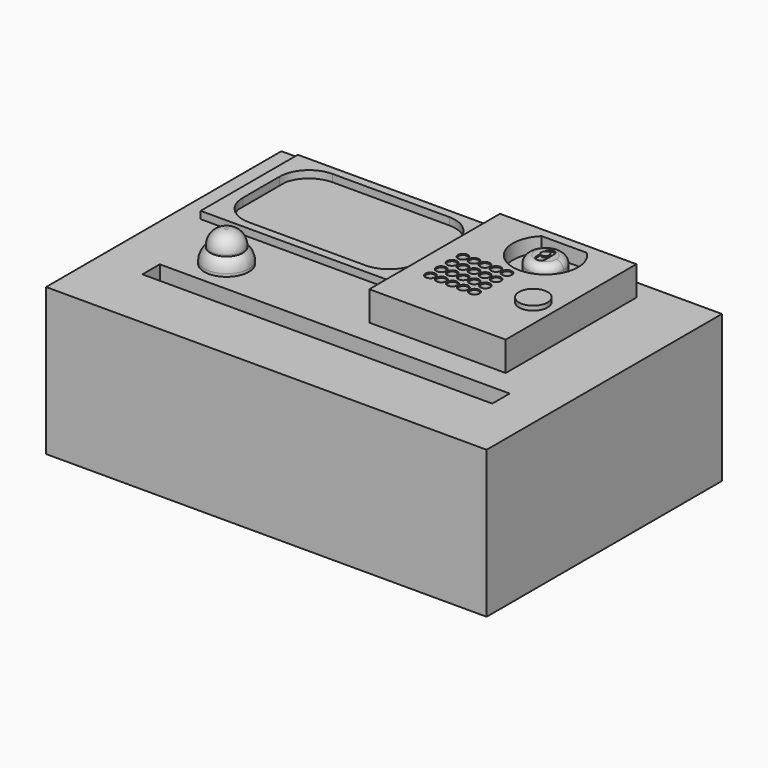
from build123d import *

# Parameters (mm, degrees)
F0_W      = 76.095610857
F0_H      = 25.4
F1_DEPTH  = 50.8
F2_W      = 60.4380872101
F2_H      = 3.7578083575
F3_DEPTH  = 63.5
F2_R      = 3.8481
F2_R_2    = 2.8067
F4_DEPTH  = 2.54
F5_DEPTH  = 5.334
F2_W_2    = 23.5645882785
F2_H_2    = 28.2227061689
F7_DEPTH  = 5.08
F8_R      = 0.7366
F8_R_2    = 0.7422011714
F8_R_3    = 0.7366978513
F9_DEPTH  = 1.1684
F10_SIZE  = 0.127
F8_R_4    = 2.4687366623
F11_DEPTH = 0.762
F12_DEPTH = 2.54
F13_DEPTH = 5.08
F14_R     = 1.27
F15_DEPTH = 0.254
F16_DEPTH = 0.254
F19_R     = 2.54
F18_W     = 34.4761237502
F18_H     = 20.9774870891
F18_W_2   = 30.3499177098
F18_H_2   = 18.0787695572
F20_DEPTH = 1.27
F21_R     = 5.08
F22_DEPTH = 2.54
F24_W     = 30.0253331661
F24_H     = 18.0815514177
F25_DEPTH = 2.54


# Not quite as in the source:
# - a fillet or chamfer that OpenCascade refuses, or shapes differently, is made with other operations: its cross-section is extruded or revolved along the edge and cut away or added
# - a feature names something its author has since deleted; it is built from what else it names


with BuildPart() as f1:
    # F0 (on Front) → F1 (new body)
    with BuildSketch(Plane.XZ):
        with Locations((38.0478054285, 12.7)):
            Rectangle(F0_W, F0_H)
    extrude(amount=F1_DEPTH)

    # F2 (on face) → F3 (cut)
    with BuildSketch(Plane.XY.offset(25.4)):
        with Locations((38.0478100851, -37.9173252732)):
            Rectangle(F2_W, F2_H)
    extrude(amount=-F3_DEPTH, mode=Mode.SUBTRACT)

    # F18 (on offset) → F22 (cut)
    with BuildSketch(Plane.XY.offset(25.4)):
        with Locations((21.1429484189, -11.8157025427)):
            Rectangle(F18_W_2, F18_H_2)
    extrude(amount=-F22_DEPTH, mode=Mode.SUBTRACT)


with BuildPart() as f4:
    # F2 (on face) → F4 (new body)
    with BuildSketch(Plane.XY.offset(25.4)):
        with Locations((14.7585952654, -30.2724912763)):
            Circle(F2_R)
        with Locations((14.7585952654, -30.2724912763)):
            Circle(F2_R_2, mode=Mode.SUBTRACT)
    extrude(amount=F4_DEPTH)

    # F6: fillet of radius 2.54 on 1 edges, made by hand

    # F6_s1 → F6_t2 (revolve, cut)
    with BuildSketch(Plane.XZ.offset(30.2724912763)):
        with BuildLine():
            ThreePointArc((18.6066952654, 25.8891957578), (18.331429687, 27.0392296703), (17.5652952654, 27.94))
            Line((17.5652952654, 27.94), (18.6066952654, 27.94))
            Line((18.6066952654, 27.94), (18.6066952654, 25.8891957578))
        make_face()
    revolve(axis=Axis((14.7585952654, -30.2724912763, 27.94), (0, 0, 1)), mode=Mode.SUBTRACT)


with BuildPart() as f5:
    # F2 (on face) → F5 (new body)
    with BuildSketch(Plane.XY.offset(25.4)):
        with Locations((14.7585952654, -30.2724912763)):
            Circle(F2_R_2)
    extrude(amount=F5_DEPTH)

    # F19
    f19_edges = [f5.edges().sort_by_distance(p)[0] for p in [
        (11.951895, -30.272491, 30.734),
    ]]
    fillet(f19_edges, radius=F19_R)


with BuildPart() as f7:
    # F2 (on face) → F7 (new body)
    with BuildSketch(Plane.XY.offset(25.4)):
        with Locations((52.3189920932, -17.5821054727)):
            Rectangle(F2_W_2, F2_H_2)
    extrude(amount=F7_DEPTH)

    # F8 (on face) → F9 (cut)
    with BuildSketch(Plane.XY.offset(30.48)):
        with Locations((44.468279928, -16.3894109428)):
            Circle(F8_R)
        with Locations((44.4501824677, -18.7166463584)):
            Circle(F8_R)
        with Locations((46.373279928, -16.3894109428)):
            Circle(F8_R)
        with Locations((48.278279928, -16.3894109428)):
            Circle(F8_R)
        with Locations((50.183279928, -16.3894109428)):
            Circle(F8_R)
        with Locations((52.088279928, -16.3894109428)):
            Circle(F8_R)
        with Locations((52.0701824677, -18.7166463584)):
            Circle(F8_R)
        with Locations((50.1651824677, -18.7166463584)):
            Circle(F8_R)
        with Locations((48.2601824677, -18.7166463584)):
            Circle(F8_R)
        with Locations((46.3551824677, -18.7166463584)):
            Circle(F8_R)
        with Locations((44.4501824677, -21.0534463584)):
            Circle(F8_R_2)
        with Locations((46.3551824677, -21.0534463584)):
            Circle(F8_R_2)
        with Locations((48.2601824677, -21.0534463584)):
            Circle(F8_R_2)
        with Locations((50.1651824677, -21.0534463584)):
            Circle(F8_R_2)
        with Locations((52.0701824677, -21.0534463584)):
            Circle(F8_R_2)
        with Locations((52.0701824677, -23.3902463584)):
            Circle(F8_R_3)
        with Locations((50.1651824677, -23.3902463584)):
            Circle(F8_R_3)
        with Locations((48.2601824677, -23.3902463584)):
            Circle(F8_R_3)
        with Locations((46.3551824677, -23.3902463584)):
            Circle(F8_R_3)
        with Locations((44.4501824677, -23.3902463584)):
            Circle(F8_R_3)
    extrude(amount=-F9_DEPTH, mode=Mode.SUBTRACT)

    # F10
    f10_edges = [f7.edges().sort_by_distance(p)[0] for p in [
        (43.73168, -16.389411, 30.48),
        (45.63668, -16.389411, 30.48),
        (47.54168, -16.389411, 29.3116),
        (49.44668, -16.389411, 29.3116),
        (45.63668, -16.389411, 29.3116),
        (43.73168, -16.389411, 29.3116),
        (47.54168, -16.389411, 30.48),
        (49.44668, -16.389411, 30.48),
        (51.35168, -16.389411, 29.3116),
        (51.35168, -16.389411, 30.48),
        (43.713582, -18.716646, 30.48),
        (43.713582, -18.716646, 29.3116),
        (45.618582, -18.716646, 30.48),
        (45.618582, -18.716646, 29.3116),
        (47.523582, -18.716646, 29.3116),
        (47.523582, -18.716646, 30.48),
        (49.428582, -18.716646, 29.3116),
        (49.428582, -18.716646, 30.48),
        (51.333582, -18.716646, 29.3116),
        (51.333582, -18.716646, 30.48),
        (51.327981, -21.053446, 29.3116),
        (51.327981, -21.053446, 30.48),
        (49.422981, -21.053446, 29.3116),
        (49.422981, -21.053446, 30.48),
        (47.517981, -21.053446, 29.3116),
        (47.517981, -21.053446, 30.48),
        (45.612981, -21.053446, 29.3116),
        (45.612981, -21.053446, 30.48),
        (43.707981, -21.053446, 29.3116),
        (43.707981, -21.053446, 30.48),
        (43.713485, -23.390246, 29.3116),
        (43.713485, -23.390246, 30.48),
        (45.618485, -23.390246, 29.3116),
        (45.618485, -23.390246, 30.48),
        (47.523485, -23.390246, 30.48),
        (47.523485, -23.390246, 29.3116),
        (49.428485, -23.390246, 29.3116),
        (49.428485, -23.390246, 30.48),
        (51.333485, -23.390246, 29.3116),
        (51.333485, -23.390246, 30.48),
    ]]
    chamfer(f10_edges, length=F10_SIZE)

    # F8 (on face) → F12 (cut)
    with BuildSketch(Plane.XY.offset(30.48)):
        with BuildLine():
            Line((56.8032637239, -5.0562927499), (49.0126051009, -5.0562927499))
            ThreePointArc((49.0126051009, -5.0562927499), (52.9079344124, -14.7297750973), (56.8032637239, -5.0562927499))
        make_face()
        with BuildLine():
            ThreePointArc((49.7954895275, -9.1378182046), (52.8933981599, -5.9961993022), (56.0205150705, -9.1087460168))
            ThreePointArc((56.0205150705, -9.1087460168), (56.020481127, -9.1232822692), (56.0203792972, -9.1378182046))
            ThreePointArc((56.0203792972, -9.1378182046), (52.9079344124, -12.2213266749), (49.7954895275, -9.1378182046))
        make_face(mode=Mode.SUBTRACT)
        with BuildLine():
            Line((52.1097108722, -9.1378182046), (49.7954895275, -9.1378182046))
            ThreePointArc((49.7954895275, -9.1378182046), (52.9079344124, -12.2213266749), (56.0203792972, -9.1378182046))
            Line((56.0203792972, -9.1378182046), (53.6705512988, -9.1378182046))
            Line((53.6705512988, -9.1378182046), (53.6705512988, -10.1698003709))
            ThreePointArc((53.6705512988, -10.1698003709), (52.8901310855, -10.8525913337), (52.1097108722, -10.1698003709))
            Line((52.1097108722, -10.1698003709), (52.1097108722, -9.1378182046))
        make_face()
        with BuildLine():
            ThreePointArc((56.0203792972, -9.1378182046), (56.020481127, -9.1232822692), (56.0205150705, -9.1087460168))
            ThreePointArc((56.0205150705, -9.1087460168), (52.8933981599, -5.9961993022), (49.7954895275, -9.1378182046))
            Line((49.7954895275, -9.1378182046), (52.1097108722, -9.1378182046))
            Line((52.1097108722, -9.1378182046), (52.1097108722, -8.0964182046))
            ThreePointArc((52.1097108722, -8.0964182046), (52.8891712862, -7.4125251355), (53.6705512988, -8.0942241475))
            Line((53.6705512988, -8.0942241475), (53.6705512988, -9.1378182046))
            Line((53.6705512988, -9.1378182046), (56.0203792972, -9.1378182046))
        make_face()
    extrude(amount=-F12_DEPTH, mode=Mode.SUBTRACT)

    # F8 (on face) → F15 (cut)
    with BuildSketch(Plane.XY.offset(30.48)):
        with BuildLine():
            Line((52.1097108722, -8.0964182046), (52.1097108722, -9.1378182046))
            Line((52.1097108722, -9.1378182046), (52.2154003667, -9.1378182046))
            ThreePointArc((52.2154003667, -9.1378182046), (52.8933951195, -8.4157545265), (53.6010784065, -9.1087460168))
            ThreePointArc((53.6010784065, -9.1087460168), (53.6009259026, -9.1232853096), (53.6004684581, -9.1378182046))
            Line((53.6004684581, -9.1378182046), (53.6705512988, -9.1378182046))
            Line((53.6705512988, -9.1378182046), (53.6705512988, -8.0942241475))
            ThreePointArc((53.6705512988, -8.0942241475), (52.8891712862, -7.4125251355), (52.1097108722, -8.0964182046))
        make_face()
        with BuildLine():
            Line((52.2154003667, -9.1378182046), (52.1097108722, -9.1378182046))
            Line((52.1097108722, -9.1378182046), (52.1097108722, -10.1698003709))
            ThreePointArc((52.1097108722, -10.1698003709), (52.8901310855, -10.8525913337), (53.6705512988, -10.1698003709))
            Line((53.6705512988, -10.1698003709), (53.6705512988, -9.1378182046))
            Line((53.6705512988, -9.1378182046), (53.6004684581, -9.1378182046))
            ThreePointArc((53.6004684581, -9.1378182046), (52.9079344124, -9.8018900109), (52.2154003667, -9.1378182046))
        make_face()
        with BuildLine():
            Line((53.6004684581, -9.1378182046), (52.2154003667, -9.1378182046))
            ThreePointArc((52.2154003667, -9.1378182046), (52.9079344124, -9.8018900109), (53.6004684581, -9.1378182046))
        make_face()
        with BuildLine():
            ThreePointArc((53.6010784065, -9.1087460168), (52.8933951195, -8.4157545265), (52.2154003667, -9.1378182046))
            Line((52.2154003667, -9.1378182046), (53.6004684581, -9.1378182046))
            ThreePointArc((53.6004684581, -9.1378182046), (53.6009259026, -9.1232853096), (53.6010784065, -9.1087460168))
        make_face()
    extrude(amount=-F15_DEPTH, mode=Mode.SUBTRACT)


with BuildPart() as f11:
    # F8 (on face) → F11 (new body)
    with BuildSketch(Plane.XY.offset(30.48)):
        with Locations((60.1860508323, -20.8426285535)):
            Circle(F8_R_4)
    extrude(amount=F11_DEPTH)


with BuildPart() as f13:
    # F8 (on face) → F13 (new body)
    with BuildSketch(Plane.XY.offset(30.48)):
        with BuildLine():
            Line((52.1097108722, -9.1378182046), (49.7954895275, -9.1378182046))
            ThreePointArc((49.7954895275, -9.1378182046), (52.9079344124, -12.2213266749), (56.0203792972, -9.1378182046))
            Line((56.0203792972, -9.1378182046), (53.6705512988, -9.1378182046))
            Line((53.6705512988, -9.1378182046), (53.6705512988, -10.1698003709))
            ThreePointArc((53.6705512988, -10.1698003709), (52.8901310855, -10.8525913337), (52.1097108722, -10.1698003709))
            Line((52.1097108722, -10.1698003709), (52.1097108722, -9.1378182046))
        make_face()
        with BuildLine():
            ThreePointArc((56.0203792972, -9.1378182046), (56.020481127, -9.1232822692), (56.0205150705, -9.1087460168))
            ThreePointArc((56.0205150705, -9.1087460168), (52.8933981599, -5.9961993022), (49.7954895275, -9.1378182046))
            Line((49.7954895275, -9.1378182046), (52.1097108722, -9.1378182046))
            Line((52.1097108722, -9.1378182046), (52.1097108722, -8.0964182046))
            ThreePointArc((52.1097108722, -8.0964182046), (52.8891712862, -7.4125251355), (53.6705512988, -8.0942241475))
            Line((53.6705512988, -8.0942241475), (53.6705512988, -9.1378182046))
            Line((53.6705512988, -9.1378182046), (56.0203792972, -9.1378182046))
        make_face()
    extrude(amount=-F13_DEPTH)

    # F14
    f14_edges = [f13.edges().sort_by_distance(p)[0] for p in [
        (49.79549, -9.079674, 30.48),
    ]]
    fillet(f14_edges, radius=F14_R)


with BuildPart() as f16:
    # F8 (on face) → F16 (new body)
    with BuildSketch(Plane.XY.offset(30.48)):
        with BuildLine():
            ThreePointArc((53.6010784065, -9.1087460168), (52.8933951195, -8.4157545265), (52.2154003667, -9.1378182046))
            Line((52.2154003667, -9.1378182046), (53.6004684581, -9.1378182046))
            ThreePointArc((53.6004684581, -9.1378182046), (53.6009259026, -9.1232853096), (53.6010784065, -9.1087460168))
        make_face()
        with BuildLine():
            Line((53.6004684581, -9.1378182046), (52.2154003667, -9.1378182046))
            ThreePointArc((52.2154003667, -9.1378182046), (52.9079344124, -9.8018900109), (53.6004684581, -9.1378182046))
        make_face()
    extrude(amount=F16_DEPTH)


with BuildPart() as f20:
    # F18 (on offset) → F20 (new body)
    with BuildSketch(Plane.XY.offset(25.4)):
        with Locations((21.1429484189, -11.8157025427)):
            Rectangle(F18_W, F18_H)
        with Locations((21.1429484189, -11.8157025427)):
            Rectangle(F18_W_2, F18_H_2, mode=Mode.SUBTRACT)
    extrude(amount=F20_DEPTH)

    # F21
    f21_edges = [f20.edges().sort_by_distance(p)[0] for p in [
        (36.317907, -2.776318, 26.035),
        (5.96799, -2.776318, 26.035),
        (36.317907, -20.855087, 26.035),
        (5.96799, -20.855087, 26.035),
    ]]
    fillet(f21_edges, radius=F21_R)


with BuildPart() as f25:
    # F24 (on offset) → F25 (new body)
    with BuildSketch(Plane.XY.offset(25.4)):
        with Locations((21.1146250367, -11.7616094649)):
            Rectangle(F24_W, F24_H)
    extrude(amount=-F25_DEPTH)


solid = Compound([f1.part, f4.part, f5.part, f7.part, f11.part, f13.part, f16.part, f20.part, f25.part])
